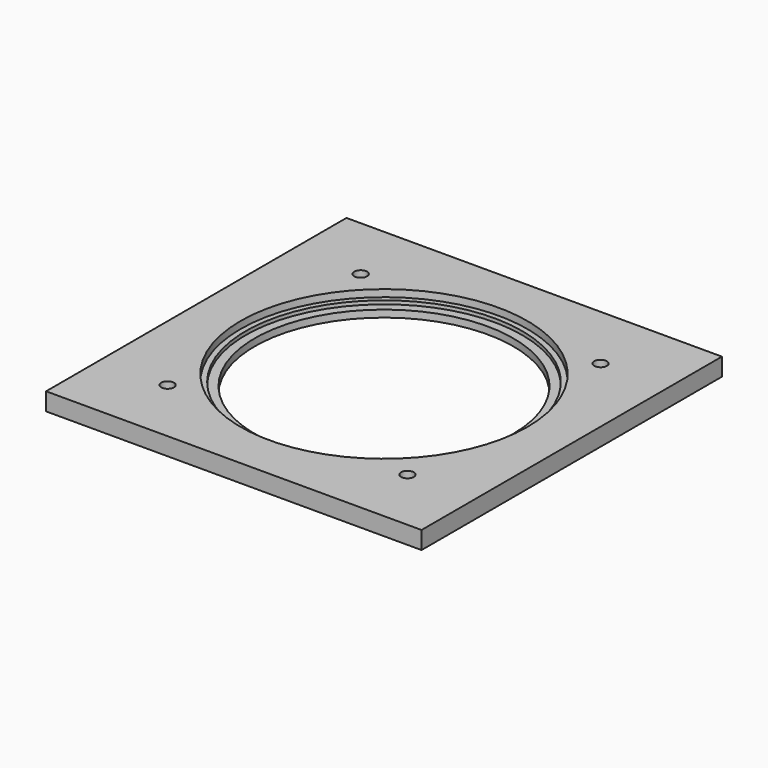
from build123d import *

# Parameters (mm, degrees)
F0_W     = 134.62
F0_H     = 134.62
F0_R     = 2.286
F0_R_2   = 51.435
F4_DEPTH = 6.35
F2_W     = 134.62
F2_H     = 134.62
F2_R     = 2.286
F2_R_2   = 49.53
F7_DEPTH = 3.81
F6_W     = 134.62
F6_H     = 134.62
F6_R     = 2.286
F6_R_2   = 46.355
F8_DEPTH = 2.54


# Not quite as in the source:
# - the program builds the solid bodies; features that only make, move or delete a surface that nothing else refers to are left out


with BuildPart() as f4:
    # F0 (on Top) → F4 (new body)
    with BuildSketch(Plane.XY):
        Rectangle(F0_W, F0_H)
        with Locations((-43.1052293811, -43.1052293811)):
            Circle(F0_R, mode=Mode.SUBTRACT)
        with Locations((43.2547706189, -43.5552815736)):
            Circle(F0_R, mode=Mode.SUBTRACT)
        with Locations((-42.9551675437, 43.2547706189)):
            Circle(F0_R, mode=Mode.SUBTRACT)
        Circle(F0_R_2, mode=Mode.SUBTRACT)
        with Locations((43.4036597586, 42.8047184264)):
            Circle(F0_R, mode=Mode.SUBTRACT)
    extrude(amount=-F4_DEPTH)

    # F2 (on offset) → F7 (join)
    with BuildSketch(Plane.XY.offset(-2.54)):
        Rectangle(F2_W, F2_H)
        with Locations((-43.1052293811, -43.1052293811)):
            Circle(F2_R, mode=Mode.SUBTRACT)
        with Locations((43.2547706189, -43.5552815736)):
            Circle(F2_R, mode=Mode.SUBTRACT)
        with Locations((-42.9551675437, 43.2547706189)):
            Circle(F2_R, mode=Mode.SUBTRACT)
        Circle(F2_R_2, mode=Mode.SUBTRACT)
        with Locations((43.4036597586, 42.8047184264)):
            Circle(F2_R, mode=Mode.SUBTRACT)
    extrude(amount=-F7_DEPTH)

    # F6 (on offset) → F8 (join)
    with BuildSketch(Plane.XY.offset(-3.81)):
        Rectangle(F6_W, F6_H)
        with Locations((-43.1052293811, -43.1052293811)):
            Circle(F6_R, mode=Mode.SUBTRACT)
        with Locations((43.2547706189, -43.5552815736)):
            Circle(F6_R, mode=Mode.SUBTRACT)
        with Locations((-42.9551675437, 43.2547706189)):
            Circle(F6_R, mode=Mode.SUBTRACT)
        Circle(F6_R_2, mode=Mode.SUBTRACT)
        with Locations((43.4036597586, 42.8047184264)):
            Circle(F6_R, mode=Mode.SUBTRACT)
    extrude(amount=-F8_DEPTH)


solid = f4.part
